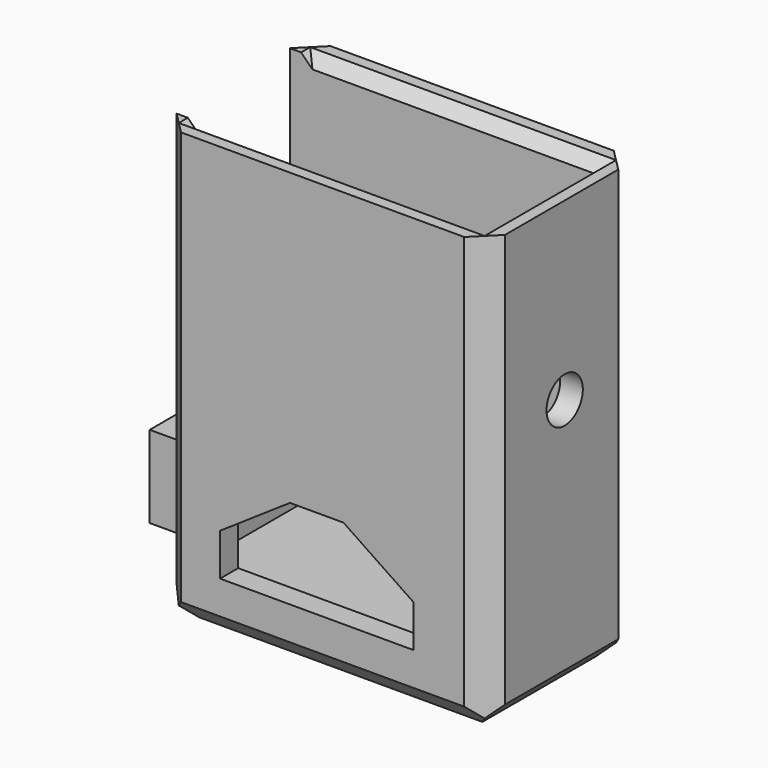
from build123d import *

# Parameters (mm, degrees)
F0_W      = 29
F0_H      = 16.5
F1_DEPTH  = 38.5
F2_T      = -2
F3_DEPTH  = 2.25
F4_SIZE   = 2
F5_SIZE   = 2
F6_SIZE   = 2
F7_SIZE   = 2
F8_SIZE   = 2
F9_SIZE   = 0.99999
F11_DEPTH = 16.501
F12_SIZE  = 2
F13_SIZE  = 2
F14_W     = 12.5
F14_H     = 2.3482141793
F15_DEPTH = 2
F16_R     = 2
F17_DEPTH = 2.001
F18_W     = 7.1378413203
F18_H     = 7.25
F18_R     = 1.1
F19_DEPTH = 4.35


# Not quite as in the source:
# - a fillet or chamfer is up to 0.001 mm smaller than in the source, because OpenCascade refuses the exact size


with BuildPart() as f1:
    # F0 (on Top) → F1 (new body)
    with BuildSketch(Plane.XY):
        with Locations((14.5, 8.25)):
            Rectangle(F0_W, F0_H)
    extrude(amount=F1_DEPTH)

    # F2
    f2_openings = [f1.faces().sort_by_distance(p)[0] for p in [
        (14.5, 8.25, 38.5),
    ]]
    offset(amount=F2_T, openings=f2_openings)

    # F3 (add): a face of the model
    f3_faces = [f1.faces().sort_by_distance(p)[0] for p in [
        (14.5, 8.25, 2),
    ]]
    extrude(f3_faces, amount=F3_DEPTH)

    # F4
    f4_edges = [f1.edges().sort_by_distance(p)[0] for p in [
        (0, 0, 19.25),
    ]]
    chamfer(f4_edges, length=F4_SIZE)

    # F5
    f5_edges = [f1.edges().sort_by_distance(p)[0] for p in [
        (0, 16.5, 19.25),
        (29, 0, 19.25),
    ]]
    chamfer(f5_edges, length=F5_SIZE)

    # F6
    f6_edges = [f1.edges().sort_by_distance(p)[0] for p in [
        (29, 16.5, 19.25),
    ]]
    chamfer(f6_edges, length=F6_SIZE)

    # F7
    f7_edges = [f1.edges().sort_by_distance(p)[0] for p in [
        (14.5, 0, 0),
    ]]
    chamfer(f7_edges, length=F7_SIZE)

    # F8
    f8_edges = [f1.edges().sort_by_distance(p)[0] for p in [
        (14.5, 16.5, 0),
    ]]
    chamfer(f8_edges, length=F8_SIZE)

    # F9 (size 1 in the source; OpenCascade refuses exactly that, so slightly less here)
    f9_edges = [f1.edges().sort_by_distance(p)[0] for p in [
        (14.5, 14.5, 38.5),
        (2, 8.25, 38.5),
        (14.5, 2, 38.5),
        (27, 8.25, 38.5),
    ]]
    chamfer(f9_edges, length=F9_SIZE)

    # F10 (on face) → F11 (cut, through all)
    with BuildSketch(Plane(origin=(0, 16.5, 0), x_dir=(-1, 0, 0), z_dir=(0, 1, 0))):
        Polygon((-16.345, 12.834), (-22.516, 8.664), (-22.516, 4.94), (-5.445, 4.94), (-5.445, 8.664), (-11.616, 12.834), align=None)
    extrude(amount=-F11_DEPTH, mode=Mode.SUBTRACT)

    # F12
    f12_edges = [f1.edges().sort_by_distance(p)[0] for p in [
        (0, 8.25, 0),
    ]]
    chamfer(f12_edges, length=F12_SIZE)

    # F13
    f13_edges = [f1.edges().sort_by_distance(p)[0] for p in [
        (29, 8.25, 0),
    ]]
    chamfer(f13_edges, length=F13_SIZE)

    # F14 (on face) → F15 (cut, through all)
    with BuildSketch(Plane(origin=(0, 0, 0), x_dir=(0, -1, 0), z_dir=(-1, 0, 0))):
        with BuildLine():
            ThreePointArc((-14.5, 28.5), (-8.25, 34.75), (-2, 28.5))
            Line((-2, 28.5), (-2, 38.5))
            Line((-2, 38.5), (-14.5, 38.5))
            Line((-14.5, 38.5), (-14.5, 28.5))
        make_face()
        with Locations((-8.25, 39.6741070896)):
            Rectangle(F14_W, F14_H)
        with BuildLine():
            Line((-14.5, 28.5), (-2, 28.5))
            ThreePointArc((-2, 28.5), (-8.25, 34.75), (-14.5, 28.5))
        make_face()
        with BuildLine():
            ThreePointArc((-11.8148919341, 23.3663808577), (-8.6306663931, 22.2616033232), (-5.335738673, 22.9710235198))
            ThreePointArc((-5.335738673, 22.9710235198), (-5.3356417901, 22.985511616), (-5.3356094956, 23))
            ThreePointArc((-5.3356094956, 23), (-8.4021264241, 26.2448164759), (-11.8148919341, 23.3663808577))
        make_face()
        with BuildLine():
            ThreePointArc((-11.8148919341, 23.3663808577), (-8.7835560201, 19.7560337281), (-5.335738673, 22.9710235198))
            ThreePointArc((-5.335738673, 22.9710235198), (-8.6306663931, 22.2616033232), (-11.8148919341, 23.3663808577))
        make_face()
        with BuildLine():
            ThreePointArc((-5.335738673, 22.9710235198), (-2.8985220129, 25.2713496081), (-2, 28.5))
            Line((-2, 28.5), (-14.5, 28.5))
            ThreePointArc((-14.5, 28.5), (-13.7881889905, 25.6032841517), (-11.8148919341, 23.3663808577))
            ThreePointArc((-11.8148919341, 23.3663808577), (-8.4021264241, 26.2448164759), (-5.3356094956, 23))
            ThreePointArc((-5.3356094956, 23), (-5.3356417901, 22.985511616), (-5.335738673, 22.9710235198))
        make_face()
    extrude(amount=-F15_DEPTH, mode=Mode.SUBTRACT)

    # F16 (on face) → F17 (cut, through all)
    with BuildSketch(Plane(origin=(27, 0, 0), x_dir=(0, -1, 0), z_dir=(-1, 0, 0))):
        with Locations((-8.5856094956, 23)):
            Circle(F16_R)
    extrude(amount=-F17_DEPTH, mode=Mode.SUBTRACT)

    # F18 (on face) → F19 (join)
    with BuildSketch(Plane(origin=(0, 0, 0), x_dir=(0, -1, 0), z_dir=(-1, 0, 0))):
        with Locations((-8.0489206601, 7.875)):
            Rectangle(F18_W, F18_H)
        with Locations((-8.25, 9)):
            Circle(F18_R, mode=Mode.SUBTRACT)
    extrude(amount=F19_DEPTH)


solid = f1.part
